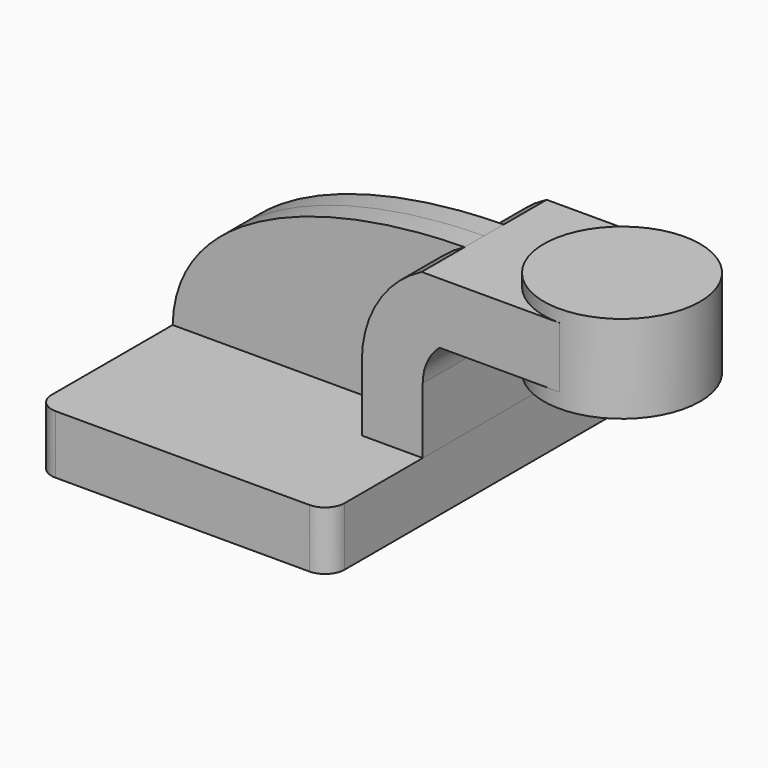
from build123d import *

# Parameters (mm, degrees)
F1_DEPTH = 63.5
F0_W     = 25.4
F0_H     = 19.7866
F2_DEPTH = 25.4
F3_DEPTH = 7.9375
F5_R     = 6.35


# Not quite as in the source:
# - a feature names something its author has since deleted; it is built from what else it names


with BuildPart() as f1:
    # F0 (on Front) → F1 (new body, symmetric)
    with BuildSketch(Plane.XZ):
        Polygon((-47.625, 9.525), (-47.625, -9.525), (47.625, -9.525), (47.625, 9.525), (27.8384, 9.525), align=None)
    extrude(amount=F1_DEPTH, both=True)

    # F5
    f5_edges = [f1.edges().sort_by_distance(p)[0] for p in [
        (47.625, -63.5, 0),
        (-47.625, -63.5, 0),
        (-47.625, 63.5, 0),
        (47.625, 63.5, 0),
    ]]
    fillet(f5_edges, radius=F5_R)


with BuildPart() as f2:
    # F0 (on Front) → F2 (new body, symmetric)
    with BuildSketch(Plane.XZ):
        with BuildLine():
            Line((27.8384, 9.525), (47.625, 9.525))
            Line((47.625, 9.525), (47.625, 30.9091658516))
            ThreePointArc((47.625, 30.9091658516), (49.0496379155, 37.4820389393), (53.0678548822, 42.8752))
            Line((53.0678548822, 42.8752), (66.675, 42.8752))
            Line((66.675, 42.8752), (66.675, 62.6618))
            Line((66.675, 62.6618), (47.2667027627, 62.6618))
            ThreePointArc((47.2667027627, 62.6618), (33.0808032049, 49.5215859226), (27.8384, 30.9091658516))
            Line((27.8384, 30.9091658516), (27.8384, 9.525))
        make_face()
        with Locations((79.375, 52.7685)):
            Rectangle(F0_W, F0_H)
    extrude(amount=F2_DEPTH, both=True)


with BuildPart() as f3:
    # F0 (on Front) → F3 (new body, symmetric)
    with BuildSketch(Plane.XZ):
        with BuildLine():
            add(Edge.make_bspline(
                [(-47.625, 9.525), (-46.8263998628, 44.964145869), (0, 62.2051432729), (47.2667027627, 62.6618)],
                knots=[0, 0, 0, 0, 108.7564010412, 108.7564010412, 108.7564010412, 108.7564010412], degree=3))
            Line((-47.625, 9.525), (27.8384, 9.525))
            Line((27.8384, 9.525), (27.8384, 30.9091658516))
            ThreePointArc((27.8384, 30.9091658516), (33.0808032049, 49.5215859226), (47.2667027627, 62.6618))
        make_face()
    extrude(amount=F3_DEPTH, both=True)


with BuildPart() as f4:
    # F0 (on Front) → F4 (revolve)
    with BuildSketch(Plane.XZ):
        Polygon((92.075, 66.675), (92.075, 62.6618), (92.075, 42.8752), (92.075, 38.1), (117.475, 38.1), (117.475, 66.675), align=None)
    revolve(axis=Axis((92.075, 0, 52.3875), (0, 0, 1)))


solid = Compound([f1.part, f2.part, f3.part, f4.part])
